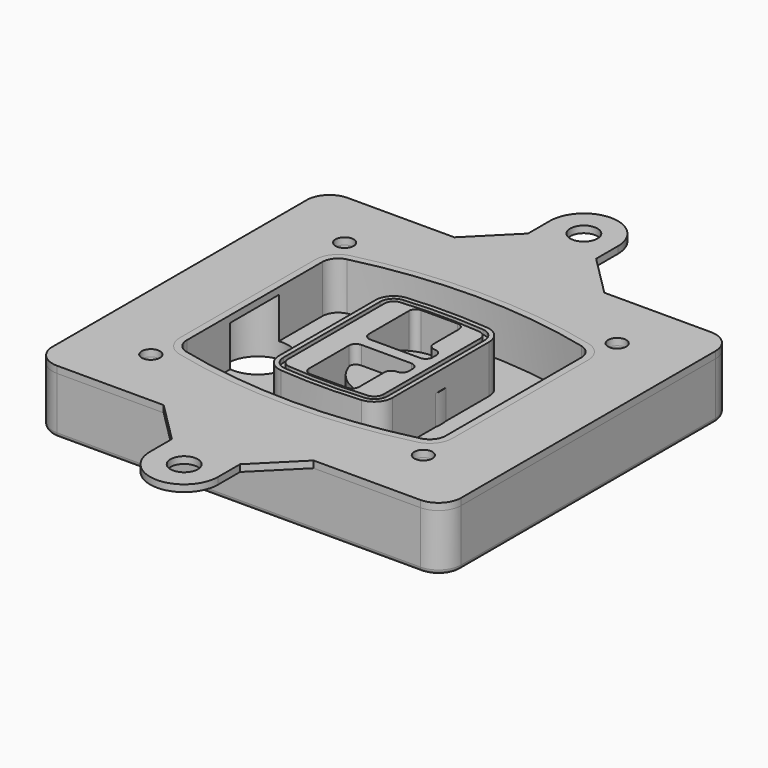
from build123d import *

# Parameters (mm, degrees)
F0_R      = 4
F1_DEPTH  = 25
F2_DEPTH  = 3
F3_DEPTH  = 18
F5_DEPTH  = 21
F6_DEPTH  = 2
F8_DEPTH  = 20
F9_DEPTH  = 16
F10_DEPTH = 25
F7_R      = 6
F7_R_2    = 4
F11_DEPTH = 6
F13_DEPTH = 9
F15_R     = 2
F16_R     = 4
F16_R_2   = 6
F17_DEPTH = 3


# Not quite as in the source:
# - a feature of the source that left no trace in its solid (it failed there, or was rolled back) is left out
# - a feature names something its author has since deleted; it is built from what else it names


with BuildPart() as f1:
    # F0 (on Top) → F1 (new body)
    with BuildSketch(Plane.XY):
        with BuildLine():
            ThreePointArc((-90, -70), (-87.0710678119, -77.0710678119), (-80, -80))
            Line((-80, -80), (80, -80))
            ThreePointArc((80, -80), (87.0710678119, -77.0710678119), (90, -70))
            Line((90, -70), (90, 70))
            ThreePointArc((90, 70), (87.0710678119, 77.0710678119), (80, 80))
            Line((80, 80), (-80, 80))
            ThreePointArc((-80, 80), (-87.0710678119, 77.0710678119), (-90, 70))
            Line((-90, 70), (-90, -70))
        make_face()
        with Locations((-60, -53.3333333333)):
            Circle(F0_R, mode=Mode.SUBTRACT)
        with Locations((60, -53.3333333333)):
            Circle(F0_R, mode=Mode.SUBTRACT)
        with Locations((-60, 53.3333333333)):
            Circle(F0_R, mode=Mode.SUBTRACT)
        with BuildLine():
            ThreePointArc((-64, 37.2990447398), (-61.0143011354, 45.9411029726), (-53.3306899286, 50.8970778549))
            ThreePointArc((-53.3306899286, 50.8970778549), (0, 57.3333333333), (53.3306899286, 50.8970778549))
            ThreePointArc((53.3306899286, 50.8970778549), (61.0143011354, 45.9411029726), (64, 37.2990447398))
            Line((64, 37.2990447398), (64, -37.2990447398))
            ThreePointArc((64, -37.2990447398), (61.0143011354, -45.9411029726), (53.3306899286, -50.8970778549))
            ThreePointArc((53.3306899286, -50.8970778549), (0, -57.3333333333), (-53.3306899286, -50.8970778549))
            ThreePointArc((-53.3306899286, -50.8970778549), (-61.0143011354, -45.9411029726), (-64, -37.2990447398))
            Line((-64, -37.2990447398), (-64, 37.2990447398))
        make_face(mode=Mode.SUBTRACT)
        with Locations((60, 53.3333333333)):
            Circle(F0_R, mode=Mode.SUBTRACT)
        with BuildLine():
            ThreePointArc((53.3306899286, 50.8970778549), (0, 57.3333333333), (-53.3306899286, 50.8970778549))
            ThreePointArc((-53.3306899286, 50.8970778549), (-61.0143011354, 45.9411029726), (-64, 37.2990447398))
            Line((-64, 37.2990447398), (-64, -37.2990447398))
            ThreePointArc((-64, -37.2990447398), (-61.0143011354, -45.9411029726), (-53.3306899286, -50.8970778549))
            ThreePointArc((-53.3306899286, -50.8970778549), (0, -57.3333333333), (53.3306899286, -50.8970778549))
            ThreePointArc((53.3306899286, -50.8970778549), (61.0143011354, -45.9411029726), (64, -37.2990447398))
            Line((64, -37.2990447398), (64, 37.2990447398))
            ThreePointArc((64, 37.2990447398), (61.0143011354, 45.9411029726), (53.3306899286, 50.8970778549))
        make_face()
        with BuildLine():
            Line((-60, -37.2990447398), (-60, 37.2990447398))
            ThreePointArc((-60, 37.2990447398), (-57.8673579538, 43.4719434775), (-52.3790642347, 47.0119255363))
            ThreePointArc((-52.3790642347, 47.0119255363), (0, 53.3333333333), (52.3790642347, 47.0119255363))
            ThreePointArc((52.3790642347, 47.0119255363), (57.8673579538, 43.4719434775), (60, 37.2990447398))
            Line((60, 37.2990447398), (60, -37.2990447398))
            ThreePointArc((60, -37.2990447398), (57.8673579538, -43.4719434775), (52.3790642347, -47.0119255363))
            ThreePointArc((52.3790642347, -47.0119255363), (0, -53.3333333333), (-52.3790642347, -47.0119255363))
            ThreePointArc((-52.3790642347, -47.0119255363), (-57.8673579538, -43.4719434775), (-60, -37.2990447398))
        make_face(mode=Mode.SUBTRACT)
        with BuildLine():
            ThreePointArc((-52.3790642347, 47.0119255363), (-57.8673579538, 43.4719434775), (-60, 37.2990447398))
            Line((-60, 37.2990447398), (-60, -37.2990447398))
            ThreePointArc((-60, -37.2990447398), (-57.8673579538, -43.4719434775), (-52.3790642347, -47.0119255363))
            ThreePointArc((-52.3790642347, -47.0119255363), (0, -53.3333333333), (52.3790642347, -47.0119255363))
            ThreePointArc((52.3790642347, -47.0119255363), (57.8673579538, -43.4719434775), (60, -37.2990447398))
            Line((60, -37.2990447398), (60, 37.2990447398))
            ThreePointArc((60, 37.2990447398), (57.8673579538, 43.4719434775), (52.3790642347, 47.0119255363))
            ThreePointArc((52.3790642347, 47.0119255363), (0, 53.3333333333), (-52.3790642347, 47.0119255363))
        make_face()
        with BuildLine():
            ThreePointArc((51.6653449643, 44.0980612973), (55.5071505677, 41.6200738562), (57, 37.2990447398))
            Line((57, 37.2990447398), (57, -37.2990447398))
            ThreePointArc((57, -37.2990447398), (55.5071505677, -41.6200738562), (51.6653449643, -44.0980612973))
            ThreePointArc((51.6653449643, -44.0980612973), (0, -50.3333333333), (-51.6653449643, -44.0980612973))
            ThreePointArc((-51.6653449643, -44.0980612973), (-55.5071505677, -41.6200738562), (-57, -37.2990447398))
            Line((-57, -37.2990447398), (-57, 37.2990447398))
            ThreePointArc((-57, 37.2990447398), (-55.5071505677, 41.6200738562), (-51.6653449643, 44.0980612973))
            ThreePointArc((-51.6653449643, 44.0980612973), (0, 50.3333333333), (51.6653449643, 44.0980612973))
        make_face(mode=Mode.SUBTRACT)
        with BuildLine():
            Line((57, -37.2990447398), (57, 37.2990447398))
            ThreePointArc((57, 37.2990447398), (55.5071505677, 41.6200738562), (51.6653449643, 44.0980612973))
            ThreePointArc((51.6653449643, 44.0980612973), (0, 50.3333333333), (-51.6653449643, 44.0980612973))
            ThreePointArc((-51.6653449643, 44.0980612973), (-55.5071505677, 41.6200738562), (-57, 37.2990447398))
            Line((-57, 37.2990447398), (-57, -37.2990447398))
            ThreePointArc((-57, -37.2990447398), (-55.5071505677, -41.6200738562), (-51.6653449643, -44.0980612973))
            ThreePointArc((-51.6653449643, -44.0980612973), (0, -50.3333333333), (51.6653449643, -44.0980612973))
            ThreePointArc((51.6653449643, -44.0980612973), (55.5071505677, -41.6200738562), (57, -37.2990447398))
        make_face()
    extrude(amount=-F1_DEPTH)

    # F0 (on Top) → F2 (join)
    with BuildSketch(Plane.XY):
        with BuildLine():
            ThreePointArc((-52.3790642347, 47.0119255363), (-57.8673579538, 43.4719434775), (-60, 37.2990447398))
            Line((-60, 37.2990447398), (-60, -37.2990447398))
            ThreePointArc((-60, -37.2990447398), (-57.8673579538, -43.4719434775), (-52.3790642347, -47.0119255363))
            ThreePointArc((-52.3790642347, -47.0119255363), (0, -53.3333333333), (52.3790642347, -47.0119255363))
            ThreePointArc((52.3790642347, -47.0119255363), (57.8673579538, -43.4719434775), (60, -37.2990447398))
            Line((60, -37.2990447398), (60, 37.2990447398))
            ThreePointArc((60, 37.2990447398), (57.8673579538, 43.4719434775), (52.3790642347, 47.0119255363))
            ThreePointArc((52.3790642347, 47.0119255363), (0, 53.3333333333), (-52.3790642347, 47.0119255363))
        make_face()
        with BuildLine():
            ThreePointArc((51.6653449643, 44.0980612973), (55.5071505677, 41.6200738562), (57, 37.2990447398))
            Line((57, 37.2990447398), (57, -37.2990447398))
            ThreePointArc((57, -37.2990447398), (55.5071505677, -41.6200738562), (51.6653449643, -44.0980612973))
            ThreePointArc((51.6653449643, -44.0980612973), (0, -50.3333333333), (-51.6653449643, -44.0980612973))
            ThreePointArc((-51.6653449643, -44.0980612973), (-55.5071505677, -41.6200738562), (-57, -37.2990447398))
            Line((-57, -37.2990447398), (-57, 37.2990447398))
            ThreePointArc((-57, 37.2990447398), (-55.5071505677, 41.6200738562), (-51.6653449643, 44.0980612973))
            ThreePointArc((-51.6653449643, 44.0980612973), (0, 50.3333333333), (51.6653449643, 44.0980612973))
        make_face(mode=Mode.SUBTRACT)
    extrude(amount=F2_DEPTH)

    # F0 (on Top) → F3 (cut)
    with BuildSketch(Plane.XY):
        with BuildLine():
            Line((57, -37.2990447398), (57, 37.2990447398))
            ThreePointArc((57, 37.2990447398), (55.5071505677, 41.6200738562), (51.6653449643, 44.0980612973))
            ThreePointArc((51.6653449643, 44.0980612973), (0, 50.3333333333), (-51.6653449643, 44.0980612973))
            ThreePointArc((-51.6653449643, 44.0980612973), (-55.5071505677, 41.6200738562), (-57, 37.2990447398))
            Line((-57, 37.2990447398), (-57, -37.2990447398))
            ThreePointArc((-57, -37.2990447398), (-55.5071505677, -41.6200738562), (-51.6653449643, -44.0980612973))
            ThreePointArc((-51.6653449643, -44.0980612973), (0, -50.3333333333), (51.6653449643, -44.0980612973))
            ThreePointArc((51.6653449643, -44.0980612973), (55.5071505677, -41.6200738562), (57, -37.2990447398))
        make_face()
    extrude(amount=-F3_DEPTH, mode=Mode.SUBTRACT)

    # F4 (on face) → F5 (join, through all)
    with BuildSketch(Plane.XY.offset(3)):
        with BuildLine():
            ThreePointArc((-25, -26.587695628), (-22.8992979869, -31.9912392117), (-17.7004291845, -34.5569740744))
            ThreePointArc((-17.7004291845, -34.5569740744), (0, -35.3333333333), (17.7004291845, -34.5569740744))
            ThreePointArc((17.7004291845, -34.5569740744), (22.8992979869, -31.9912392117), (25, -26.587695628))
            Line((25, -26.587695628), (25, 26.587695628))
            ThreePointArc((25, 26.587695628), (22.8992979869, 31.9912392117), (17.7004291845, 34.5569740744))
            ThreePointArc((17.7004291845, 34.5569740744), (0, 35.3333333333), (-17.7004291845, 34.5569740744))
            ThreePointArc((-17.7004291845, 34.5569740744), (-22.8992979869, 31.9912392117), (-25, 26.587695628))
            Line((-25, 26.587695628), (-25, -26.587695628))
        make_face()
        with BuildLine():
            ThreePointArc((17.5253218884, 32.5646544628), (21.4244734902, 30.6403533158), (23, 26.587695628))
            Line((23, 26.587695628), (23, -26.587695628))
            ThreePointArc((23, -26.587695628), (21.4244734902, -30.6403533158), (17.5253218884, -32.5646544628))
            ThreePointArc((17.5253218884, -32.5646544628), (0, -33.3333333333), (-17.5253218884, -32.5646544628))
            ThreePointArc((-17.5253218884, -32.5646544628), (-21.4244734902, -30.6403533158), (-23, -26.587695628))
            Line((-23, -26.587695628), (-23, 26.587695628))
            ThreePointArc((-23, 26.587695628), (-21.4244734902, 30.6403533158), (-17.5253218884, 32.5646544628))
            ThreePointArc((-17.5253218884, 32.5646544628), (0, 33.3333333333), (17.5253218884, 32.5646544628))
        make_face(mode=Mode.SUBTRACT)
        with BuildLine():
            Line((23, -26.587695628), (23, 26.587695628))
            ThreePointArc((23, 26.587695628), (21.4244734902, 30.6403533158), (17.5253218884, 32.5646544628))
            ThreePointArc((17.5253218884, 32.5646544628), (0, 33.3333333333), (-17.5253218884, 32.5646544628))
            ThreePointArc((-17.5253218884, 32.5646544628), (-21.4244734902, 30.6403533158), (-23, 26.587695628))
            Line((-23, 26.587695628), (-23, -26.587695628))
            ThreePointArc((-23, -26.587695628), (-21.4244734902, -30.6403533158), (-17.5253218884, -32.5646544628))
            ThreePointArc((-17.5253218884, -32.5646544628), (0, -33.3333333333), (17.5253218884, -32.5646544628))
            ThreePointArc((17.5253218884, -32.5646544628), (21.4244734902, -30.6403533158), (23, -26.587695628))
        make_face()
        with BuildLine():
            ThreePointArc((17.3502145923, 30.5723348512), (19.9496489934, 29.2894674198), (21, 26.587695628))
            Line((21, 26.587695628), (21, -26.587695628))
            ThreePointArc((21, -26.587695628), (19.9496489934, -29.2894674198), (17.3502145923, -30.5723348512))
            ThreePointArc((17.3502145923, -30.5723348512), (0, -31.3333333333), (-17.3502145923, -30.5723348512))
            ThreePointArc((-17.3502145923, -30.5723348512), (-19.9496489934, -29.2894674198), (-21, -26.587695628))
            Line((-21, -26.587695628), (-21, 26.587695628))
            ThreePointArc((-21, 26.587695628), (-19.9496489934, 29.2894674198), (-17.3502145923, 30.5723348512))
            ThreePointArc((-17.3502145923, 30.5723348512), (0, 31.3333333333), (17.3502145923, 30.5723348512))
        make_face(mode=Mode.SUBTRACT)
        with BuildLine():
            Line((21, -26.587695628), (21, 26.587695628))
            ThreePointArc((21, 26.587695628), (19.9496489934, 29.2894674198), (17.3502145923, 30.5723348512))
            ThreePointArc((17.3502145923, 30.5723348512), (0, 31.3333333333), (-17.3502145923, 30.5723348512))
            ThreePointArc((-17.3502145923, 30.5723348512), (-19.9496489934, 29.2894674198), (-21, 26.587695628))
            Line((-21, 26.587695628), (-21, -26.587695628))
            ThreePointArc((-21, -26.587695628), (-19.9496489934, -29.2894674198), (-17.3502145923, -30.5723348512))
            ThreePointArc((-17.3502145923, -30.5723348512), (0, -31.3333333333), (17.3502145923, -30.5723348512))
            ThreePointArc((17.3502145923, -30.5723348512), (19.9496489934, -29.2894674198), (21, -26.587695628))
        make_face()
        with BuildLine():
            Line((-8, -2.5), (14, -2.5))
            ThreePointArc((14, -2.5), (16.1213203436, -3.3786796564), (17, -5.5))
            Line((17, -5.5), (17, -7.5))
            ThreePointArc((17, -7.5), (16.1213203436, -9.6213203436), (14, -10.5))
            ThreePointArc((14, -10.5), (11.8786796564, -11.3786796564), (11, -13.5))
            Line((11, -13.5), (11, -27.5))
            ThreePointArc((11, -27.5), (10.1213203436, -29.6213203436), (8, -30.5))
            Line((8, -30.5), (-8, -30.5))
            ThreePointArc((-8, -30.5), (-10.1213203436, -29.6213203436), (-11, -27.5))
            Line((-11, -27.5), (-11, -5.5))
            ThreePointArc((-11, -5.5), (-10.1213203436, -3.3786796564), (-8, -2.5))
        make_face(mode=Mode.SUBTRACT)
        with BuildLine():
            ThreePointArc((-8, 2.5), (-10.1213203436, 3.3786796564), (-11, 5.5))
            Line((-11, 5.5), (-11, 27.5))
            ThreePointArc((-11, 27.5), (-10.1213203436, 29.6213203436), (-8, 30.5))
            Line((-8, 30.5), (8, 30.5))
            ThreePointArc((8, 30.5), (10.1213203436, 29.6213203436), (11, 27.5))
            Line((11, 27.5), (11, 13.5))
            ThreePointArc((11, 13.5), (11.8786796564, 11.3786796564), (14, 10.5))
            ThreePointArc((14, 10.5), (16.1213203436, 9.6213203436), (17, 7.5))
            Line((17, 7.5), (17, 5.5))
            ThreePointArc((17, 5.5), (16.1213203436, 3.3786796564), (14, 2.5))
            Line((14, 2.5), (-8, 2.5))
        make_face(mode=Mode.SUBTRACT)
    extrude(amount=-F5_DEPTH)

    # F4 (on face) → F6 (cut)
    with BuildSketch(Plane.XY.offset(3)):
        with BuildLine():
            Line((23, -26.587695628), (23, 26.587695628))
            ThreePointArc((23, 26.587695628), (21.4244734902, 30.6403533158), (17.5253218884, 32.5646544628))
            ThreePointArc((17.5253218884, 32.5646544628), (0, 33.3333333333), (-17.5253218884, 32.5646544628))
            ThreePointArc((-17.5253218884, 32.5646544628), (-21.4244734902, 30.6403533158), (-23, 26.587695628))
            Line((-23, 26.587695628), (-23, -26.587695628))
            ThreePointArc((-23, -26.587695628), (-21.4244734902, -30.6403533158), (-17.5253218884, -32.5646544628))
            ThreePointArc((-17.5253218884, -32.5646544628), (0, -33.3333333333), (17.5253218884, -32.5646544628))
            ThreePointArc((17.5253218884, -32.5646544628), (21.4244734902, -30.6403533158), (23, -26.587695628))
        make_face()
        with BuildLine():
            ThreePointArc((17.3502145923, 30.5723348512), (19.9496489934, 29.2894674198), (21, 26.587695628))
            Line((21, 26.587695628), (21, -26.587695628))
            ThreePointArc((21, -26.587695628), (19.9496489934, -29.2894674198), (17.3502145923, -30.5723348512))
            ThreePointArc((17.3502145923, -30.5723348512), (0, -31.3333333333), (-17.3502145923, -30.5723348512))
            ThreePointArc((-17.3502145923, -30.5723348512), (-19.9496489934, -29.2894674198), (-21, -26.587695628))
            Line((-21, -26.587695628), (-21, 26.587695628))
            ThreePointArc((-21, 26.587695628), (-19.9496489934, 29.2894674198), (-17.3502145923, 30.5723348512))
            ThreePointArc((-17.3502145923, 30.5723348512), (0, 31.3333333333), (17.3502145923, 30.5723348512))
        make_face(mode=Mode.SUBTRACT)
    extrude(amount=-F6_DEPTH, mode=Mode.SUBTRACT)

    # F7 (on face) → F8 (join)
    with BuildSketch(Plane(origin=(0, 0, -25), x_dir=(1, 0, 0), z_dir=(0, 0, -1))):
        with BuildLine():
            ThreePointArc((-6.71157564, 0), (6.7567035675, 13.4682792075), (20.224982775, 0))
            Line((20.224982775, 0), (25.224982775, 0))
            ThreePointArc((25.224982775, 0), (6.7567035675, 18.4682792075), (-11.71157564, 0))
            Line((-11.71157564, 0), (-6.71157564, 0))
        make_face()
        with BuildLine():
            Line((-6.71157564, 0), (20.224982775, 0))
            ThreePointArc((20.224982775, 0), (6.7567035675, 13.4682792075), (-6.71157564, 0))
        make_face()
        with BuildLine():
            ThreePointArc((-6.71157564, 0), (6.7567035675, -13.4682792075), (20.224982775, 0))
            Line((20.224982775, 0), (-6.71157564, 0))
        make_face()
        with BuildLine():
            Line((25.224982775, 0), (20.224982775, 0))
            ThreePointArc((20.224982775, 0), (6.7567035675, -13.4682792075), (-6.71157564, 0))
            Line((-6.71157564, 0), (-11.71157564, 0))
            ThreePointArc((-11.71157564, 0), (6.7567035675, -18.4682792075), (25.224982775, 0))
        make_face()
    extrude(amount=-F8_DEPTH)

    # F7 (on face) → F9 (cut)
    with BuildSketch(Plane(origin=(0, 0, -25), x_dir=(1, 0, 0), z_dir=(0, 0, -1))):
        with BuildLine():
            Line((-6.71157564, 0), (20.224982775, 0))
            ThreePointArc((20.224982775, 0), (6.7567035675, 13.4682792075), (-6.71157564, 0))
        make_face()
        with BuildLine():
            ThreePointArc((-6.71157564, 0), (6.7567035675, -13.4682792075), (20.224982775, 0))
            Line((20.224982775, 0), (-6.71157564, 0))
        make_face()
    extrude(amount=-F9_DEPTH, mode=Mode.SUBTRACT)

    # F7 (on face) → F10 (cut)
    with BuildSketch(Plane(origin=(0, 0, -25), x_dir=(1, 0, 0), z_dir=(0, 0, -1))):
        with BuildLine():
            Line((-69.0318229325, 0), (-42.0952645175, 0))
            ThreePointArc((-42.0952645175, 0), (-55.563543725, 13.4682792075), (-69.0318229325, 0))
        make_face()
        with BuildLine():
            ThreePointArc((-69.0318229325, 0), (-55.563543725, -13.4682792075), (-42.0952645175, 0))
            Line((-42.0952645175, 0), (-69.0318229325, 0))
        make_face()
    extrude(amount=-F10_DEPTH, mode=Mode.SUBTRACT)

    # F7 (on face) → F11 (cut)
    with BuildSketch(Plane(origin=(0, 0, -25), x_dir=(1, 0, 0), z_dir=(0, 0, -1))):
        with Locations((60, -53.3333333333)):
            Circle(F7_R)
        with Locations((60, -53.3333333333)):
            Circle(F7_R_2, mode=Mode.SUBTRACT)
        with Locations((-60, -53.3333333333)):
            Circle(F7_R)
        with Locations((-60, -53.3333333333)):
            Circle(F7_R_2, mode=Mode.SUBTRACT)
        with Locations((-60, 53.3333333333)):
            Circle(F7_R)
        with Locations((-60, 53.3333333333)):
            Circle(F7_R_2, mode=Mode.SUBTRACT)
        with Locations((60, 53.3333333333)):
            Circle(F7_R)
        with Locations((60, 53.3333333333)):
            Circle(F7_R_2, mode=Mode.SUBTRACT)
    extrude(amount=-F11_DEPTH, mode=Mode.SUBTRACT)

    # F12 (on face) → F13 (cut, through all)
    with BuildSketch(Plane(origin=(0, 0, -9), x_dir=(1, 0, 0), z_dir=(0, 0, -1))):
        with BuildLine():
            ThreePointArc((20.224982775, 0), (20.1663399806, 1.2554664788), (19.9909222755, 2.5))
            Line((19.9909222755, 2.5), (14, 2.5))
            ThreePointArc((14, 2.5), (16.1213203436, 3.3786796564), (17, 5.5))
            Line((17, 5.5), (17, 7.5))
            ThreePointArc((17, 7.5), (16.1213203436, 9.6213203436), (14, 10.5))
            ThreePointArc((14, 10.5), (12.1627255951, 11.1284134507), (11.0951631559, 12.750384826))
            ThreePointArc((11.0951631559, 12.750384826), (11.0476113807, 12.7664660322), (11, 12.7823698976))
            Line((11, 12.7823698976), (11, -12.7823698976))
            ThreePointArc((11, -12.7823698976), (11.0476113807, -12.7664660322), (11.0951631559, -12.750384826))
            ThreePointArc((11.0951631559, -12.750384826), (12.1627255951, -11.1284134507), (14, -10.5))
            ThreePointArc((14, -10.5), (16.1213203436, -9.6213203436), (17, -7.5))
            Line((17, -7.5), (17, -5.5))
            ThreePointArc((17, -5.5), (16.1213203436, -3.3786796564), (14, -2.5))
            Line((14, -2.5), (19.9909222755, -2.5))
            ThreePointArc((19.9909222755, -2.5), (20.1663399806, -1.2554664788), (20.224982775, 0))
        make_face()
    extrude(amount=F13_DEPTH, mode=Mode.SUBTRACT)

    # F15
    f15_edges = [f1.edges().sort_by_distance(p)[0] for p in [
        (0, -80, -25),
        (-87.071068, -77.071068, -25),
        (-90, 0, -25),
        (-87.071068, 77.071068, -25),
        (87.071068, -77.071068, -25),
        (0, 80, -25),
        (90, 0, -25),
        (87.071068, 77.071068, -25),
    ]]
    fillet(f15_edges, radius=F15_R)


with BuildPart() as f17:
    # F16 (on face) → F17 (new body, through all)
    with BuildSketch(Plane.XY):
        with BuildLine():
            Line((-90, 70), (-90, -70))
            ThreePointArc((-90, -70), (-87.0710678119, -77.0710678119), (-80, -80))
            Line((-80, -80), (-33, -80))
            Line((-33, -80), (33, -80))
            Line((33, -80), (80, -80))
            ThreePointArc((80, -80), (87.0710678119, -77.0710678119), (90, -70))
            Line((90, -70), (90, 70))
            ThreePointArc((90, 70), (87.0710678119, 77.0710678119), (80, 80))
            Line((80, 80), (33, 80))
            Line((33, 80), (-33, 80))
            Line((-33, 80), (-80, 80))
            ThreePointArc((-80, 80), (-87.0710678119, 77.0710678119), (-90, 70))
        make_face()
        with Locations((-60, -53.3333333333)):
            Circle(F16_R, mode=Mode.SUBTRACT)
        with Locations((60, -53.3333333333)):
            Circle(F16_R, mode=Mode.SUBTRACT)
        with Locations((-60, 53.3333333333)):
            Circle(F16_R, mode=Mode.SUBTRACT)
        with BuildLine():
            ThreePointArc((52.3790642347, -47.0119255363), (0, -53.3333333333), (-52.3790642347, -47.0119255363))
            ThreePointArc((-52.3790642347, -47.0119255363), (-57.8673579538, -43.4719434775), (-60, -37.2990447398))
            Line((-60, -37.2990447398), (-60, 37.2990447398))
            ThreePointArc((-60, 37.2990447398), (-57.8673579538, 43.4719434775), (-52.3790642347, 47.0119255363))
            ThreePointArc((-52.3790642347, 47.0119255363), (0, 53.3333333333), (52.3790642347, 47.0119255363))
            ThreePointArc((52.3790642347, 47.0119255363), (57.8673579538, 43.4719434775), (60, 37.2990447398))
            Line((60, 37.2990447398), (60, -37.2990447398))
            ThreePointArc((60, -37.2990447398), (57.8673579538, -43.4719434775), (52.3790642347, -47.0119255363))
        make_face(mode=Mode.SUBTRACT)
        with Locations((60, 53.3333333333)):
            Circle(F16_R, mode=Mode.SUBTRACT)
        with BuildLine():
            Line((33, -80), (-33, -80))
            Line((-33, -80), (-15, -98))
            Line((-15, -98), (-15, -110))
            ThreePointArc((-15, -110), (0, -125), (15, -110))
            Line((15, -110), (15, -98))
            Line((15, -98), (33, -80))
        make_face()
        with Locations((0, -110)):
            Circle(F16_R_2, mode=Mode.SUBTRACT)
        with BuildLine():
            Line((-15, 98), (-33, 80))
            Line((-33, 80), (33, 80))
            Line((33, 80), (15, 98))
            Line((15, 98), (15, 110))
            ThreePointArc((15, 110), (0, 125), (-15, 110))
            Line((-15, 110), (-15, 98))
        make_face()
        with Locations((0, 110)):
            Circle(F16_R_2, mode=Mode.SUBTRACT)
    extrude(amount=F17_DEPTH)


solid = Compound([f1.part, f17.part])
